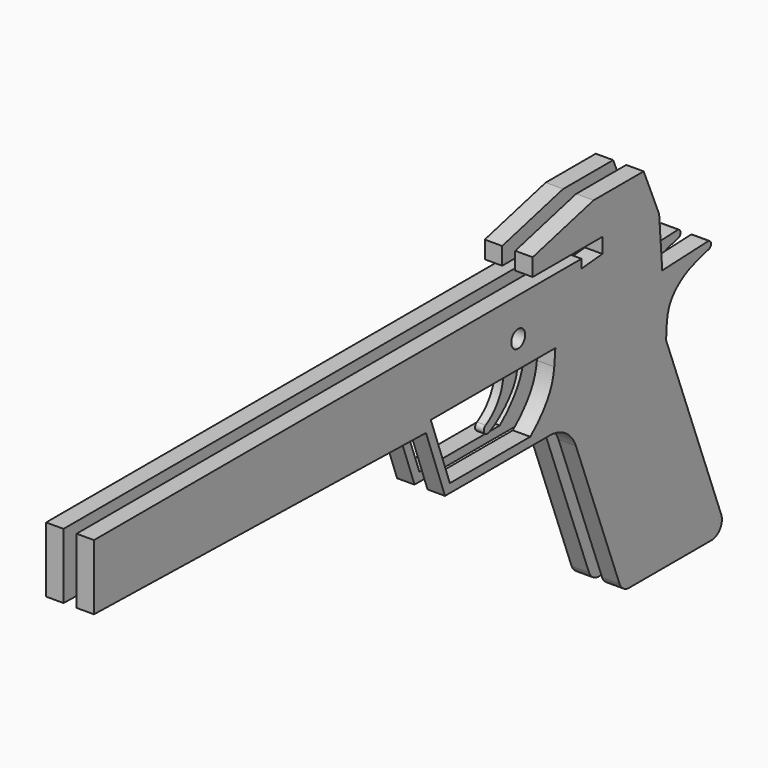
from build123d import *

# Parameters (mm, degrees)
F1_START = -0.5
F0_R     = 2
F0_R_2   = 1
F1_DEPTH = 2
F2_DEPTH = 4


# Not quite as in the source:
# - ends of sketch curves that miss each other by under 0.0002 mm in the source are joined
# - the dataset's text gives a spline's control points without its knots; the knots are read off the source's solid
# - a feature names something its author has since deleted; it is built from what else it names


with BuildPart() as f1:
    # F0 (on Right) → F1 (new body)
    with BuildSketch(Plane.YZ.offset(F1_START)):
        with BuildLine():
            ThreePointArc((74.2699354887, -13.6226043105), (74.5256304067, -14.3029139587), (74.7312395212, -14.9999978852))
            Line((74.7312395212, -14.9999978852), (79.5344771551, -14.9999978852))
            add(Edge.make_bspline(
                [(79.5344771551, -14.9999978852), (79.833759811, -14.3420916762), (80.3656146055, -13.855022927), (81.3782960176, -13.6226043105)],
                knots=[0.8797014903, 0.8797014903, 0.8797014903, 0.8797014903, 1, 1, 1, 1], degree=3))
            Line((81.3782960176, -13.6226043105), (91.4055867413, -10.9148137206))
            Line((91.4055867413, -10.9148137206), (95.2672621608, -9.8719988018))
            Line((95.2672621608, -9.8719988018), (95.2672621608, -7.9305966889))
            Line((95.2672621608, -7.9305966889), (95.2672621608, -3.9305966889))
            Line((95.2672621608, -3.9305966889), (95.2672621608, -1.989194576))
            Line((95.2672621608, -1.989194576), (89.7907053864, -2.4806121155))
            Line((89.7907053864, -2.4806121155), (89.7907053864, -5.4806121155))
            Line((89.7907053864, -5.4806121155), (84.7907053864, -5.4806121155))
            Line((84.7907053864, -5.4806121155), (82.4494448697, -3.1393515989))
            Line((82.4494448697, -3.1393515989), (69.5844688412, -4.2937402278))
            Line((69.5844688412, -4.2937402278), (68.2608369428, -4.2937402278))
            ThreePointArc((68.2608369428, -4.2937402278), (63.5964049015, -8.9581722692), (68.2608369428, -13.6226043105))
            Line((68.2608369428, -13.6226043105), (74.2699354887, -13.6226043105))
        make_face()
        with Locations((73.6394673586, -8.7706744671)):
            Circle(F0_R, mode=Mode.SUBTRACT)
        with BuildLine():
            ThreePointArc((74.7312395212, -14.9999978852), (74.229250114, -21.4306402993), (69.9054296146, -26.2170514299))
            ThreePointArc((69.9054296146, -26.2170514299), (69.4234887038, -26.8405376944), (69.5427737838, -27.6194941971))
            add(Edge.make_bspline(
                [(69.5427737838, -27.6194941971), (69.7756231299, -27.9934208955), (70.8908571939, -28.846881775), (79.88515612, -22.0379378106), (78.9360042075, -16.3156072614), (79.5344771551, -14.9999978852)],
                knots=[0.0751310014, 0.0751310014, 0.0751310014, 0.0751310014, 0.1909888597, 0.6391415971, 0.8797014903, 0.8797014903, 0.8797014903, 0.8797014903], degree=3))
            Line((79.5344771551, -14.9999978852), (74.7312395212, -14.9999978852))
        make_face()
        with BuildLine():
            Line((95.2672621608, -3.9305966889), (95.2672621608, -7.9305966889))
            Line((95.2672621608, -7.9305966889), (97.2672621608, -7.9305966889))
            ThreePointArc((97.2672621608, -7.9305966889), (99.2672621608, -5.9305966889), (97.2672621608, -3.9305966889))
            Line((97.2672621608, -3.9305966889), (95.2672621608, -3.9305966889))
        make_face()
        with Locations((97.2672621608, -5.9305966889)):
            Circle(F0_R_2, mode=Mode.SUBTRACT)
    extrude(amount=-F1_DEPTH)


with BuildPart() as f2:
    # F0 (on Right) → F2 (new body)
    with BuildSketch(Plane.YZ):
        with BuildLine():
            ThreePointArc((82.7154165104, -32.0100596195), (87.2584865329, -33.4251894787), (90.194298045, -37.1699309267))
            Line((90.194298045, -37.1699309267), (102.7124142253, -70.1337568918))
            ThreePointArc((102.7124142253, -70.1337568918), (103.8133435424, -71.5380349348), (105.5169948008, -72.068708632))
            Line((105.5169948008, -72.068708632), (129.0989228233, -72.068708632))
            ThreePointArc((129.0989228233, -72.068708632), (131.5682491261, -70.7723598904), (131.9035033988, -68.0036603722))
            Line((131.9035033988, -68.0036603722), (116.0789003285, -26.3328966518))
            add(Edge.make_bspline(
                [(116.0789003285, -26.3328966518), (116.1564016078, -24.1501429386), (116.2971797879, -20.1785641936), (119.0310238282, -16.7283649073), (122.8788302042, -14.3416877179), (126.3069431811, -13.450153948), (128.1059980392, -12.9797337577)],
                knots=[0, 0, 0, 0, 0.2769497136, 0.5036740855, 0.738714159, 1, 1, 1, 1], degree=3))
            ThreePointArc((128.1059980392, -12.9797337577), (128.982509952, -12.1032218449), (128.1059980392, -11.2267099321))
            Line((128.1059980392, -11.2267099321), (114.9739147732, -11.7841614367))
            Line((114.9739147732, -11.7841614367), (114.0789003285, 0))
            Line((114.0789003285, 0), (109.6443608403, 10.4085551575))
            Line((109.6443608403, 10.4085551575), (95.2672621608, 10.4085551575))
            Line((95.2672621608, 10.4085551575), (77.7900875211, 6))
            Line((77.7900875211, 6), (77.7900875211, 2))
            Line((77.7900875211, 2), (97.7900875211, 2))
            Line((97.7900875211, 2), (97.7900875211, 0))
            Line((97.7900875211, 0), (97.7900875211, -1.4616133168))
            Line((97.7900875211, -1.4616133168), (91.7900875211, -2))
            Line((91.7900875211, -2), (91.7900875211, 0))
            Line((91.7900875211, 0), (-48.0964966012, 0))
            Line((-48.0964966012, 0), (-48.0964966012, -15))
            Line((-48.0964966012, -15), (47.1827716724, -17.0506781676))
            Line((47.1827716724, -17.0506781676), (52.6275412439, -32.0100596195))
            Line((52.6275412439, -32.0100596195), (82.7154165104, -32.0100596195))
        make_face()
        with BuildLine():
            Line((48.5647406346, -14.9999978852), (74.7312395212, -14.9999978852))
            ThreePointArc((74.7312395212, -14.9999978852), (74.5256304067, -14.3029139587), (74.2699354887, -13.6226043105))
            Line((74.2699354887, -13.6226043105), (68.2608369428, -13.6226043105))
            ThreePointArc((68.2608369428, -13.6226043105), (63.5964049015, -8.9581722692), (68.2608369428, -4.2937402278))
            Line((68.2608369428, -4.2937402278), (69.5844688412, -4.2937402278))
            Line((69.5844688412, -4.2937402278), (82.4494448697, -3.1393515989))
            Line((82.4494448697, -3.1393515989), (84.7907053864, -5.4806121155))
            Line((84.7907053864, -5.4806121155), (89.7907053864, -5.4806121155))
            Line((89.7907053864, -5.4806121155), (89.7907053864, -2.4806121155))
            Line((89.7907053864, -2.4806121155), (95.2672621608, -1.989194576))
            Line((95.2672621608, -1.989194576), (95.2672621608, -3.9305966889))
            Line((95.2672621608, -3.9305966889), (97.2672621608, -3.9305966889))
            ThreePointArc((97.2672621608, -3.9305966889), (99.2672621608, -5.9305966889), (97.2672621608, -7.9305966889))
            Line((97.2672621608, -7.9305966889), (95.2672621608, -7.9305966889))
            Line((95.2672621608, -7.9305966889), (95.2672621608, -9.8719988018))
            Line((95.2672621608, -9.8719988018), (95.7886696202, -11.8028365115))
            Line((95.7886696202, -11.8028365115), (91.9269942007, -12.8456514304))
            Line((91.9269942007, -12.8456514304), (91.4055867413, -10.9148137206))
            Line((91.4055867413, -10.9148137206), (81.3782960176, -13.6226043105))
            add(Edge.make_bspline(
                [(79.5344771551, -14.9999978852), (79.833759811, -14.3420916762), (80.3656146055, -13.855022927), (81.3782960176, -13.6226043105)],
                knots=[0.8797014903, 0.8797014903, 0.8797014903, 0.8797014903, 1, 1, 1, 1], degree=3))
            Line((79.5344771551, -14.9999978852), (84.2950418591, -14.9999978852))
            Line((84.2950418591, -14.9999978852), (83.986338858, -18.6614259073))
            add(Edge.make_bspline(
                [(77.0986897784, -30.0000272336), (77.4741298849, -29.6976374668), (78.3368077115, -28.960094006), (79.6638223749, -27.6571775431), (80.7998106474, -26.3257545652), (81.6427583036, -25.1541637131), (82.2327671194, -24.2151704071), (82.6797224931, -23.3743926577), (83.002030475, -22.6607865386), (83.1867359511, -22.1955964224), (83.3220738815, -21.8126055157), (83.4441699526, -21.4374057344), (83.5752904919, -20.9792524975), (83.7019603463, -20.4522364549), (83.8361720396, -19.7834574031), (83.9254022758, -19.1835780723), (83.97287916, -18.7827266699), (83.986338858, -18.6614259073)],
                knots=[0.3840308553, 0.3840308553, 0.3840308553, 0.3840308553, 0.4248462567, 0.4779520388, 0.5310578209, 0.5576107119, 0.584163603, 0.610716494, 0.6239929395, 0.6372693851, 0.6439076078, 0.6505458306, 0.6638222761, 0.6770987216, 0.6903751672, 0.7169280582, 0.7291158391, 0.7291158391, 0.7291158391, 0.7291158391], degree=3))
            Line((77.0986897784, -30.0000272336), (54.0242941486, -29.9999978852))
            Line((54.0242941486, -29.9999978852), (48.5647406346, -14.9999978852))
        make_face(mode=Mode.SUBTRACT)
        with BuildLine():
            ThreePointArc((74.2699354887, -13.6226043105), (74.5256304067, -14.3029139587), (74.7312395212, -14.9999978852))
            Line((74.7312395212, -14.9999978852), (79.5344771551, -14.9999978852))
            add(Edge.make_bspline(
                [(79.5344771551, -14.9999978852), (79.833759811, -14.3420916762), (80.3656146055, -13.855022927), (81.3782960176, -13.6226043105)],
                knots=[0.8797014903, 0.8797014903, 0.8797014903, 0.8797014903, 1, 1, 1, 1], degree=3))
            Line((81.3782960176, -13.6226043105), (91.4055867413, -10.9148137206))
            Line((91.4055867413, -10.9148137206), (95.2672621608, -9.8719988018))
            Line((95.2672621608, -9.8719988018), (95.2672621608, -7.9305966889))
            Line((95.2672621608, -7.9305966889), (95.2672621608, -3.9305966889))
            Line((95.2672621608, -3.9305966889), (95.2672621608, -1.989194576))
            Line((95.2672621608, -1.989194576), (89.7907053864, -2.4806121155))
            Line((89.7907053864, -2.4806121155), (89.7907053864, -5.4806121155))
            Line((89.7907053864, -5.4806121155), (84.7907053864, -5.4806121155))
            Line((84.7907053864, -5.4806121155), (82.4494448697, -3.1393515989))
            Line((82.4494448697, -3.1393515989), (69.5844688412, -4.2937402278))
            Line((69.5844688412, -4.2937402278), (68.2608369428, -4.2937402278))
            ThreePointArc((68.2608369428, -4.2937402278), (63.5964049015, -8.9581722692), (68.2608369428, -13.6226043105))
            Line((68.2608369428, -13.6226043105), (74.2699354887, -13.6226043105))
        make_face()
        with Locations((73.6394673586, -8.7706744671)):
            Circle(F0_R, mode=Mode.SUBTRACT)
        with BuildLine():
            Line((95.2672621608, -3.9305966889), (95.2672621608, -7.9305966889))
            Line((95.2672621608, -7.9305966889), (97.2672621608, -7.9305966889))
            ThreePointArc((97.2672621608, -7.9305966889), (99.2672621608, -5.9305966889), (97.2672621608, -3.9305966889))
            Line((97.2672621608, -3.9305966889), (95.2672621608, -3.9305966889))
        make_face()
        with Locations((97.2672621608, -5.9305966889)):
            Circle(F0_R_2, mode=Mode.SUBTRACT)
        Polygon((95.2672621608, -9.8719988018), (91.4055867413, -10.9148137206), (91.9269942007, -12.8456514304), (95.7886696202, -11.8028365115), align=None)
        with Locations((97.2672621608, -5.9305966889)):
            Circle(F0_R_2)
    extrude(amount=F2_DEPTH)


with BuildPart() as f4_1:
    # F4: instance of F2
    add(f2.part.mirror(Plane.YZ.offset(-1.5)))


solid = Compound([f1.part, f2.part, f4_1.part])
